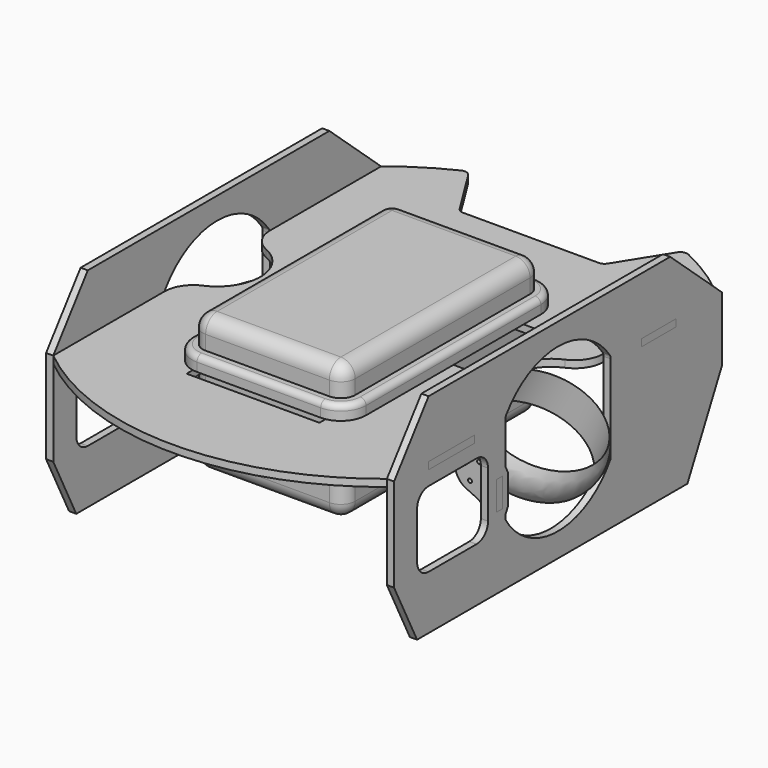
from build123d import *

# Parameters (mm, degrees)
F2_DEPTH  = 6.35
F4_DEPTH  = 82.55
F5_R      = 12.7
F9_W      = 50.8
F9_H      = 6.35
F9_W_2    = 38.1
F11_DEPTH = 6.35
F12_DEPTH = 25.4
F13_W     = 6.35
F13_H     = 25.4
F14_DEPTH = 25.4
F16_DEPTH = 12.7
F18_DEPTH = 25.4
F19_R     = 5.08
F20_R     = 12.7
F22_R     = 1.75
F22_W     = 6.35
F22_H     = 25.4
F23_DEPTH = 6.35


with BuildPart() as f2:
    # F1 (on Top) → F2 (new body)
    with BuildSketch(Plane.XY):
        with BuildLine():
            ThreePointArc((-100.401004912, 210.6532013468), (-124.7462343217, 197.2143758643), (-147.32, 180.975))
            Line((-147.32, 180.975), (-147.32, 130.175))
            Line((-147.32, 130.175), (-153.67, 130.175))
            Line((-153.67, 130.175), (-153.67, 92.075))
            Line((-153.67, 92.075), (-147.32, 92.075))
            Line((-147.32, 92.075), (-147.32, 58.1987113259))
            ThreePointArc((-147.32, 58.1987113259), (-143.171164674, 44.2865583653), (-132.08, 34.9192267956))
            ThreePointArc((-132.08, 34.9192267956), (-109.22, 0), (-132.08, -34.9192267956))
            ThreePointArc((-132.08, -34.9192267956), (-143.171164674, -44.2865583653), (-147.32, -58.1987113259))
            Line((-147.32, -58.1987113259), (-147.32, -92.075))
            Line((-147.32, -92.075), (-153.67, -92.075))
            Line((-153.67, -92.075), (-153.67, -142.875))
            Line((-153.67, -142.875), (-147.32, -142.875))
            Line((-147.32, -142.875), (-147.32, -180.975))
            ThreePointArc((-147.32, -180.975), (0, -233.3562363105), (147.32, -180.975))
            Line((147.32, -180.975), (147.32, -142.875))
            Line((147.32, -142.875), (153.67, -142.875))
            Line((153.67, -142.875), (153.67, -92.075))
            Line((153.67, -92.075), (147.32, -92.075))
            Line((147.32, -92.075), (147.32, -58.1987113259))
            ThreePointArc((147.32, -58.1987113259), (143.171164674, -44.2865583653), (132.08, -34.9192267956))
            ThreePointArc((132.08, -34.9192267956), (109.22, 0), (132.08, 34.9192267956))
            ThreePointArc((132.08, 34.9192267956), (143.171164674, 44.2865583653), (147.32, 58.1987113259))
            Line((147.32, 58.1987113259), (147.32, 92.075))
            Line((147.32, 92.075), (153.67, 92.075))
            Line((153.67, 92.075), (153.67, 130.175))
            Line((153.67, 130.175), (147.32, 130.175))
            Line((147.32, 130.175), (147.32, 180.975))
            ThreePointArc((147.32, 180.975), (124.7462343217, 197.2143758643), (100.401004912, 210.6532013468))
            ThreePointArc((100.401004912, 210.6532013468), (95.8914144419, 211.0171284406), (92.2841422163, 208.2864808567))
            Line((92.2841422163, 208.2864808567), (65.3653167069, 165.2163600417))
            ThreePointArc((65.3653167069, 165.2163600417), (63.0588076571, 163.0278735548), (59.9805274764, 162.2318533107))
            Line((59.9805274764, 162.2318533107), (0, 162.2318533107))
            Line((0, 162.2318533107), (-59.9805274764, 162.2318533107))
            ThreePointArc((-59.9805274764, 162.2318533107), (-63.0588076571, 163.0278735548), (-65.3653167069, 165.2163600417))
            Line((-65.3653167069, 165.2163600417), (-92.2841422163, 208.2864808567))
            ThreePointArc((-92.2841422163, 208.2864808567), (-95.8914144419, 211.0171284406), (-100.401004912, 210.6532013468))
        make_face()
        with BuildLine():
            Line((-67.31, 58.0857905605), (-67.31, 83.4857905605))
            ThreePointArc((-67.31, 83.4857905605), (-65.4501280605, 87.9759186211), (-60.96, 89.8357905605))
            Line((-60.96, 89.8357905605), (-23.114, 89.8357905605))
            Line((-23.114, 89.8357905605), (-23.114, 112.0607905605))
            ThreePointArc((-23.114, 112.0607905605), (-21.2541280605, 116.5509186211), (-16.764, 118.4107905605))
            Line((-16.764, 118.4107905605), (16.764, 118.4107905605))
            ThreePointArc((16.764, 118.4107905605), (21.2541280605, 116.5509186211), (23.114, 112.0607905605))
            Line((23.114, 112.0607905605), (23.114, 89.8357905605))
            Line((23.114, 89.8357905605), (60.96, 89.8357905605))
            ThreePointArc((60.96, 89.8357905605), (65.4501280605, 87.9759186211), (67.31, 83.4857905605))
            Line((67.31, 83.4857905605), (67.31, 58.0857905605))
            Line((67.31, 58.0857905605), (86.614, 58.0857905605))
            Line((86.614, 58.0857905605), (86.614, 26.8437905605))
            Line((86.614, 26.8437905605), (89.535, 26.8437905605))
            ThreePointArc((89.535, 26.8437905605), (94.0251280605, 24.9839186211), (95.885, 20.4937905605))
            Line((95.885, 20.4937905605), (95.885, -13.0342094395))
            ThreePointArc((95.885, -13.0342094395), (94.0251280605, -17.5243375), (89.535, -19.3842094395))
            Line((89.535, -19.3842094395), (67.31, -19.3842094395))
            Line((67.31, -19.3842094395), (67.31, -122.2542094395))
            ThreePointArc((67.31, -122.2542094395), (65.4501280605, -126.7443375), (60.96, -128.6042094395))
            Line((60.96, -128.6042094395), (58.674, -128.6042094395))
            Line((58.674, -128.6042094395), (58.674, -144.6062094395))
            Line((58.674, -144.6062094395), (-58.674, -144.6062094395))
            Line((-58.674, -144.6062094395), (-58.674, -128.6042094395))
            Line((-58.674, -128.6042094395), (-60.96, -128.6042094395))
            ThreePointArc((-60.96, -128.6042094395), (-65.4501280605, -126.7443375), (-67.31, -122.2542094395))
            Line((-67.31, -122.2542094395), (-67.31, -19.3842094395))
            Line((-67.31, -19.3842094395), (-89.535, -19.3842094395))
            ThreePointArc((-89.535, -19.3842094395), (-94.0251280605, -17.5243375), (-95.885, -13.0342094395))
            Line((-95.885, -13.0342094395), (-95.885, 20.4937905605))
            ThreePointArc((-95.885, 20.4937905605), (-94.0251280605, 24.9839186211), (-89.535, 26.8437905605))
            Line((-89.535, 26.8437905605), (-86.614, 26.8437905605))
            Line((-86.614, 26.8437905605), (-86.614, 58.0857905605))
            Line((-86.614, 58.0857905605), (-67.31, 58.0857905605))
        make_face(mode=Mode.SUBTRACT)
    extrude(amount=F2_DEPTH)


with BuildPart() as f4:
    # F3 (on face) → F4 (new body)
    with BuildSketch(Plane.XY.offset(6.35)):
        with BuildLine():
            Line((-67.31, -19.3842094395), (-67.31, -115.9042094395))
            ThreePointArc((-67.31, -115.9042094395), (-63.5902561211, -124.8844655605), (-54.61, -128.6042094395))
            Line((-54.61, -128.6042094395), (54.61, -128.6042094395))
            ThreePointArc((54.61, -128.6042094395), (63.5902561211, -124.8844655605), (67.31, -115.9042094395))
            Line((67.31, -115.9042094395), (67.31, -19.3842094395))
            Line((67.31, -19.3842094395), (67.31, 58.0857905605))
            Line((67.31, 58.0857905605), (67.31, 77.1357905605))
            ThreePointArc((67.31, 77.1357905605), (63.5902561211, 86.1160466816), (54.61, 89.8357905605))
            Line((54.61, 89.8357905605), (23.114, 89.8357905605))
            Line((23.114, 89.8357905605), (-23.114, 89.8357905605))
            Line((-23.114, 89.8357905605), (-54.61, 89.8357905605))
            ThreePointArc((-54.61, 89.8357905605), (-63.5902561211, 86.1160466816), (-67.31, 77.1357905605))
            Line((-67.31, 77.1357905605), (-67.31, 58.0857905605))
            Line((-67.31, 58.0857905605), (-67.31, -19.3842094395))
        make_face()
    extrude(amount=-F4_DEPTH)

    # F5
    f5_edges = [f4.edges().sort_by_distance(p)[0] for p in [
        (-67.31, -19.384209, -76.2),
    ]]
    fillet(f5_edges, radius=F5_R)

    # F15 (on face) → F16 (join)
    with BuildSketch(Plane.XY.offset(6.35)):
        with BuildLine():
            Line((54.61, 99.3607905605), (-54.61, 99.3607905605))
            ThreePointArc((-54.61, 99.3607905605), (-70.3254482119, 92.8512387724), (-76.835, 77.1357905605))
            Line((-76.835, 77.1357905605), (-76.835, -115.9042094395))
            ThreePointArc((-76.835, -115.9042094395), (-70.3254482119, -131.6196576513), (-54.61, -138.1292094395))
            Line((-54.61, -138.1292094395), (54.61, -138.1292094395))
            ThreePointArc((54.61, -138.1292094395), (70.3254482119, -131.6196576513), (76.835, -115.9042094395))
            Line((76.835, -115.9042094395), (76.835, 77.1357905605))
            ThreePointArc((76.835, 77.1357905605), (70.3254482119, 92.8512387724), (54.61, 99.3607905605))
        make_face()
        with BuildLine():
            Line((-54.61, 89.8357905605), (54.61, 89.8357905605))
            ThreePointArc((54.61, 89.8357905605), (63.5902561211, 86.1160466816), (67.31, 77.1357905605))
            Line((67.31, 77.1357905605), (67.31, -115.9042094395))
            ThreePointArc((67.31, -115.9042094395), (63.5902561211, -124.8844655605), (54.61, -128.6042094395))
            Line((54.61, -128.6042094395), (-54.61, -128.6042094395))
            ThreePointArc((-54.61, -128.6042094395), (-63.5902561211, -124.8844655605), (-67.31, -115.9042094395))
            Line((-67.31, -115.9042094395), (-67.31, 77.1357905605))
            ThreePointArc((-67.31, 77.1357905605), (-63.5902561211, 86.1160466816), (-54.61, 89.8357905605))
        make_face(mode=Mode.SUBTRACT)
        with BuildLine():
            ThreePointArc((67.31, 77.1357905605), (63.5902561211, 86.1160466816), (54.61, 89.8357905605))
            Line((54.61, 89.8357905605), (-54.61, 89.8357905605))
            ThreePointArc((-54.61, 89.8357905605), (-63.5902561211, 86.1160466816), (-67.31, 77.1357905605))
            Line((-67.31, 77.1357905605), (-67.31, -115.9042094395))
            ThreePointArc((-67.31, -115.9042094395), (-63.5902561211, -124.8844655605), (-54.61, -128.6042094395))
            Line((-54.61, -128.6042094395), (54.61, -128.6042094395))
            ThreePointArc((54.61, -128.6042094395), (63.5902561211, -124.8844655605), (67.31, -115.9042094395))
            Line((67.31, -115.9042094395), (67.31, 77.1357905605))
        make_face()
    extrude(amount=F16_DEPTH)

    # F17 (on face) → F18 (join)
    with BuildSketch(Plane.XY.offset(19.05)):
        with BuildLine():
            ThreePointArc((67.31, 77.1357905605), (63.5902561211, 86.1160466816), (54.61, 89.8357905605))
            Line((54.61, 89.8357905605), (-54.61, 89.8357905605))
            ThreePointArc((-54.61, 89.8357905605), (-63.5902561211, 86.1160466816), (-67.31, 77.1357905605))
            Line((-67.31, 77.1357905605), (-67.31, -115.9042094395))
            ThreePointArc((-67.31, -115.9042094395), (-63.5902561211, -124.8844655605), (-54.61, -128.6042094395))
            Line((-54.61, -128.6042094395), (54.61, -128.6042094395))
            ThreePointArc((54.61, -128.6042094395), (63.5902561211, -124.8844655605), (67.31, -115.9042094395))
            Line((67.31, -115.9042094395), (67.31, 77.1357905605))
        make_face()
    extrude(amount=F18_DEPTH)

    # F19
    f19_edges = [f4.edges().sort_by_distance(p)[0] for p in [
        (-76.835, -19.384209, 19.05),
        (0, 99.360791, 19.05),
        (70.325448, 92.851239, 19.05),
        (-70.325448, 92.851239, 19.05),
        (76.835, -19.384209, 19.05),
        (70.325448, -131.619658, 19.05),
        (-70.325448, -131.619658, 19.05),
        (0, -138.129209, 19.05),
    ]]
    fillet(f19_edges, radius=F19_R)

    # F20
    f20_edges = [f4.edges().sort_by_distance(p)[0] for p in [
        (-67.31, -19.384209, 44.45),
        (63.590256, 86.116047, 44.45),
        (0, 89.835791, 44.45),
        (-63.590256, 86.116047, 44.45),
        (-63.590256, -124.884466, 44.45),
        (0, -128.604209, 44.45),
        (63.590256, -124.884466, 44.45),
        (67.31, -19.384209, 44.45),
    ]]
    fillet(f20_edges, radius=F20_R)


with BuildPart() as f7:
    # F6 (on Front) → F7 (revolve)
    with BuildSketch(Plane.XZ):
        with BuildLine():
            ThreePointArc((171.1633479906, -73.0371398399), (182.0302747225, -60.5883465321), (184.5814778009, -44.2618676015))
            Line((184.5814778009, -44.2618676015), (171.1633479906, -73.0371398399))
        make_face()
    revolve(axis=Axis((133.7439001072, 0, -39.0905163845), (0.4226182617, 0, 0.906307787)))


with BuildPart() as f8_1:
    # F8: instance of F7
    add(f7.part.mirror(Plane.YZ))


with BuildPart() as f11:
    # F9 (on face) → F11 (new body)
    with BuildSketch(Plane.YZ.offset(153.67)):
        Polygon((-142.875, 57.15), (-180.975, 6.35), (-180.975, -76.2), (-155.575, -127), (142.875, -127), (180.975, -50.8), (180.975, 6.35), (123.825, 57.15), align=None)
        with Locations((-117.475, 3.175)):
            Rectangle(F9_W, F9_H, mode=Mode.SUBTRACT)
        with BuildLine():
            ThreePointArc((-57.0573070128, 8.0389898897), (0, 37.8107648032), (57.0573070128, 8.0389898897))
            ThreePointArc((57.0573070128, 8.0389898897), (57.9066434241, 6.310438469), (58.1987113259, 4.4067686725))
            Line((58.1987113259, 4.4067686725), (58.1987113259, -73.025))
            ThreePointArc((58.1987113259, -73.025), (0, -105.8976504417), (-58.1987113259, -73.025))
            Line((-58.1987113259, -73.025), (-58.1987113259, -69.85))
            Line((-58.1987113259, -69.85), (-55.6940986631, -64.8407746743))
            ThreePointArc((-55.6940986631, -64.8407746743), (-55.1935802428, -63.4598993884), (-55.0237113259, -62.0009683429))
            Line((-55.0237113259, -62.0009683429), (-55.0237113259, -39.5990316571))
            ThreePointArc((-55.0237113259, -39.5990316571), (-55.1935802428, -38.1401006116), (-55.6940986631, -36.7592253257))
            Line((-55.6940986631, -36.7592253257), (-57.5283239888, -33.0907746743))
            ThreePointArc((-57.5283239888, -33.0907746743), (-58.0288424091, -31.7098993884), (-58.1987113259, -30.2509683429))
            Line((-58.1987113259, -30.2509683429), (-58.1987113259, 0))
            Line((-58.1987113259, 0), (-58.1987113259, 4.4067686725))
            ThreePointArc((-58.1987113259, 4.4067686725), (-57.9066434241, 6.310438469), (-57.0573070128, 8.0389898897))
        make_face(mode=Mode.SUBTRACT)
        with Locations((111.125, 3.175)):
            Rectangle(F9_W_2, F9_H, mode=Mode.SUBTRACT)
    extrude(amount=-F11_DEPTH)

    # F10 (on face) → F12 (cut)
    with BuildSketch(Plane.YZ.offset(153.67)):
        with BuildLine():
            ThreePointArc((-77.2487113259, -25.4), (-80.9684552049, -16.4197438789), (-89.9487113259, -12.7))
            Line((-89.9487113259, -12.7), (-142.875, -12.7))
            ThreePointArc((-142.875, -12.7), (-151.8552561211, -16.4197438789), (-155.575, -25.4))
            Line((-155.575, -25.4), (-155.575, -66.675))
            ThreePointArc((-155.575, -66.675), (-151.8552561211, -75.6552561211), (-142.875, -79.375))
            Line((-142.875, -79.375), (-89.9487113259, -79.375))
            ThreePointArc((-89.9487113259, -79.375), (-80.9684552049, -75.6552561211), (-77.2487113259, -66.675))
            Line((-77.2487113259, -66.675), (-77.2487113259, -25.4))
        make_face()
    extrude(amount=-F12_DEPTH, mode=Mode.SUBTRACT)

    # F13 (on face) → F14 (cut)
    with BuildSketch(Plane.YZ.offset(153.67)):
        with Locations((-64.5487113259, -50.8)):
            Rectangle(F13_W, F13_H)
    extrude(amount=-F14_DEPTH, mode=Mode.SUBTRACT)


with BuildPart() as f21_1:
    # F21: instance of F11
    add(f11.part.mirror(Plane.YZ))

    # F24: F23 across plane


with BuildPart() as f23:
    # F22 (on face) → F23 (new body)
    with BuildSketch(Plane.XZ.offset(61.3737113259)):
        with BuildLine():
            Line((147.32, -63.5), (147.32, -38.1))
            Line((147.32, -38.1), (147.32, -25.1480988926))
            Line((147.32, -25.1480988926), (141.5089313758, -22.4383530911))
            ThreePointArc((141.5089313758, -22.4383530911), (118.4646670192, -30.8257793875), (126.8520933156, -53.870043744))
            Line((126.8520933156, -53.870043744), (136.0098887186, -58.1403938723))
            ThreePointArc((136.0098887186, -58.1403938723), (139.7127920094, -60.7610548445), (142.2584136361, -64.515940628))
            Line((142.2584136361, -64.515940628), (147.32, -75.9666264057))
            Line((147.32, -75.9666264057), (147.32, -63.5))
        make_face()
        with Locations((130.1550734026, -46.7867800891)):
            Circle(F22_R, mode=Mode.SUBTRACT)
        with Locations((125.5479306742, -34.1287594745)):
            Circle(F22_R, mode=Mode.SUBTRACT)
        with Locations((142.8130940172, -42.1796373606)):
            Circle(F22_R, mode=Mode.SUBTRACT)
        with Locations((138.2059512888, -29.521616746)):
            Circle(F22_R, mode=Mode.SUBTRACT)
        with Locations((150.495, -50.8)):
            Rectangle(F22_W, F22_H)
    extrude(amount=F23_DEPTH)


with BuildPart() as f21_1_1:
    add(f21_1.part)
    add(f23.part.mirror(Plane.YZ))


solid = Compound([f2.part, f4.part, f7.part, f8_1.part, f11.part, f23.part, f21_1_1.part])
